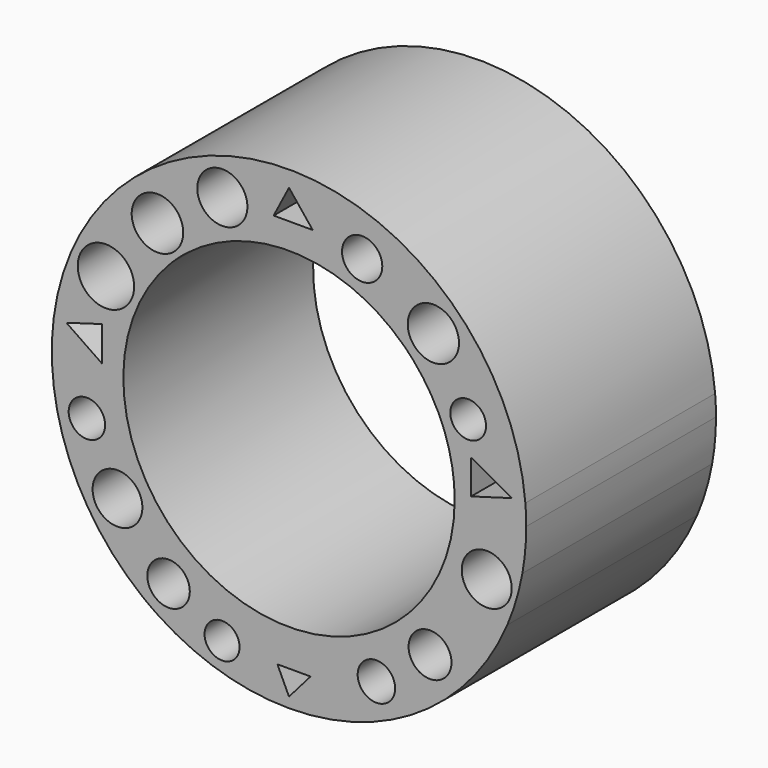
from build123d import *

# Parameters (mm, degrees)
F0_R     = 2.8256485239
F0_R_2   = 3.5765465122
F0_R_3   = 2.7439429232
F0_R_4   = 3.3466336439
F0_R_5   = 3.4276298102
F0_R_6   = 3.6294104123
F0_R_7   = 2.635041669
F0_R_8   = 2.702327646
F0_R_9   = 2.972249944
F0_R_10  = 2.6404432644
F0_R_11  = 2.6241403427
F0_R_12  = 2.7159497561
F0_R_13  = 2.2390207397
F0_R_14  = 2.2607819858
F0_R_15  = 1.9741758504
F0_R_16  = 2.1219308593
F0_R_17  = 1.8827842167
F0_R_18  = 1.845321618
F0_R_19  = 1.9213841029
F1_DEPTH = 25


with BuildPart() as f1:
    # F0 (on Front) → F1 (new body)
    with BuildSketch(Plane.XZ):
        with BuildLine():
            ThreePointArc((24.5960952758, -4.4757230907), (24.8988190673, -2.2469555075), (25, 0))
            ThreePointArc((25, 0), (24.9769503507, 1.073289886), (24.9078439057, 2.1446006555))
            ThreePointArc((24.9078439057, 2.1446006555), (0.5208838947, 24.9945730103), (-24.7968706797, 3.1804409279))
            ThreePointArc((-24.7968706797, 3.1804409279), (-23.1514874221, -9.4344385176), (-15.5110739298, -19.6062894384))
            ThreePointArc((-15.5110739298, -19.6062894384), (-13.7709472228, -14.2438804489), (-9.2095510788, -17.5570566207))
            ThreePointArc((-9.2095510788, -17.5570566207), (-10.6398306506, -20.3713740635), (-13.7563172666, -20.8749547368))
            ThreePointArc((-13.7563172666, -20.8749547368), (-7.1807427047, -23.9465432622), (0, -25))
            ThreePointArc((0, -25), (13.7903970721, -20.8524566561), (23.0050925772, -9.7859958876))
            ThreePointArc((23.0050925772, -9.7859958876), (16.860220208, -5.0514647504), (24.5960952758, -4.4757230907))
        make_face()
        with Locations((-7.0527321659, -21.0157949477)):
            Circle(F0_R, mode=Mode.SUBTRACT)
        with Locations((-18.0755164474, -11.404263787)):
            Circle(F0_R_2, mode=Mode.SUBTRACT)
        with Locations((-21.2986432016, -5.0265877508)):
            Circle(F0_R_3, mode=Mode.SUBTRACT)
        Polygon((4.266737029, -20.0934484601), (0, -25), (-2.6190390345, -20.0934484601), align=None, mode=Mode.SUBTRACT)
        with Locations((9.209163487, -19.5164699107)):
            Circle(F0_R_4, mode=Mode.SUBTRACT)
        with Locations((14.8604605347, -15.1914991438)):
            Circle(F0_R_5, mode=Mode.SUBTRACT)
        with BuildLine():
            Line((-18.9121421427, -0.7938772906), (-24.7968706797, 3.1804409279))
            Line((-24.7968706797, 3.1804409279), (-19.3468905014, 5.0684465431))
            ThreePointArc((-19.3468905014, 5.0684465431), (-21.9186154294, 11.469459375), (-15.5548330751, 8.8069401681))
            ThreePointArc((-15.5548330751, 8.8069401681), (-16.5182971087, 6.3016908172), (-18.9121421427, 5.0875890061))
            Line((-18.9121421427, 5.0875890061), (-18.9121421427, -0.7938772906))
        make_face(mode=Mode.SUBTRACT)
        with Locations((-7.0253848098, 20.105432719)):
            Circle(F0_R_6, mode=Mode.SUBTRACT)
        with BuildLine():
            Line((19.5046194307, 4.8279847044), (24.9078439057, 2.1446006555))
            Line((24.9078439057, 2.1446006555), (18.717167899, 0))
            Line((18.717167899, 0), (18.717167899, 4.7704775792))
            ThreePointArc((18.717167899, 4.7704775792), (17.4488389654, 5.1069570809), (16.4242905584, 5.9268212774))
            ThreePointArc((16.4242905584, 5.9268212774), (17.1998275024, 3.0083990244), (17.4609430101, 0))
            ThreePointArc((17.4609430101, 0), (-6.6059492578, -16.1631050607), (-12.4625227562, 12.2298837833))
            ThreePointArc((-12.4625227562, 12.2298837833), (-16.8312529103, 17.4566617233), (-10.3065616702, 15.4987508431))
            ThreePointArc((-10.3065616702, 15.4987508431), (-10.4242678564, 14.5913936768), (-10.7695943307, 13.7441030538))
            ThreePointArc((-10.7695943307, 13.7441030538), (-2.5101792072, 17.2795697617), (6.4137999623, 16.2403109836))
            ThreePointArc((6.4137999623, 16.2403109836), (5.9393579148, 21.9051948536), (10.9397131516, 19.2010402679))
            ThreePointArc((10.9397131516, 19.2010402679), (9.558784183, 16.551960716), (6.5962795119, 16.1670537638))
            ThreePointArc((6.5962795119, 16.1670537638), (9.4231129686, 14.6999820674), (11.9364463054, 12.7438526513))
            ThreePointArc((11.9364463054, 12.7438526513), (14.1879258767, 18.3986934482), (19.0337079573, 14.7156538442))
            ThreePointArc((19.0337079573, 14.7156538442), (17.0365778867, 11.3571292026), (13.1320353046, 11.5080050208))
            ThreePointArc((13.1320353046, 11.5080050208), (14.5572332623, 9.6421725015), (15.7192265164, 7.6020029287))
            ThreePointArc((15.7192265164, 7.6020029287), (18.7083751896, 11.1226574982), (22.0615752041, 7.9468004405))
            ThreePointArc((22.0615752041, 7.9468004405), (21.3406257649, 5.9303038237), (19.5046194307, 4.8279847044))
        make_face(mode=Mode.SUBTRACT)
        Polygon((3.975788597, 19.6694843471), (-2.6190390345, 19.6694843471), (0, 24.2276750505), align=None, mode=Mode.SUBTRACT)
        with BuildLine():
            ThreePointArc((23.0050925772, -9.7859958876), (23.9482362722, -7.1750943862), (24.5960952758, -4.4757230907))
            ThreePointArc((24.5960952758, -4.4757230907), (16.860220208, -5.0514647504), (23.0050925772, -9.7859958876))
        make_face()
        with Locations((20.8382867277, -6.2433271669)):
            Circle(F0_R_7, mode=Mode.SUBTRACT)
        with BuildLine():
            ThreePointArc((11.9364463054, 12.7438526513), (12.5494630323, 12.1406551883), (13.1320353046, 11.5080050208))
            ThreePointArc((13.1320353046, 11.5080050208), (17.0365778867, 11.3571292026), (19.0337079573, 14.7156538442))
            ThreePointArc((19.0337079573, 14.7156538442), (14.1879258767, 18.3986934482), (11.9364463054, 12.7438526513))
        make_face()
        with Locations((15.2111686766, 14.7156538442)):
            Circle(F0_R_8, mode=Mode.SUBTRACT)
        with BuildLine():
            ThreePointArc((-15.5548330751, 8.8069401681), (-21.9186154294, 11.469459375), (-19.3468905014, 5.0684465431))
            Line((-19.3468905014, 5.0684465431), (-18.9121421427, 5.2190539427))
            Line((-18.9121421427, 5.2190539427), (-18.9121421427, 5.0875890061))
            ThreePointArc((-18.9121421427, 5.0875890061), (-16.5182971087, 6.3016908172), (-15.5548330751, 8.8069401681))
        make_face()
        with Locations((-19.2937050015, 8.8069401681)):
            Circle(F0_R_9, mode=Mode.SUBTRACT)
        with Locations((-7.0253848098, 20.105432719)):
            Circle(F0_R_6)
        with Locations((-7.0253848098, 20.105432719)):
            Circle(F0_R_10, mode=Mode.SUBTRACT)
        with Locations((-18.0755164474, -11.404263787)):
            Circle(F0_R_2)
        with Locations((-18.0755164474, -11.404263787)):
            Circle(F0_R_11, mode=Mode.SUBTRACT)
        with BuildLine():
            ThreePointArc((-10.3065616702, 15.4987508431), (-16.8312529103, 17.4566617233), (-12.4625227562, 12.2298837833))
            ThreePointArc((-12.4625227562, 12.2298837833), (-11.6407057812, 13.0145495395), (-10.7695943307, 13.7441030538))
            ThreePointArc((-10.7695943307, 13.7441030538), (-10.4242678564, 14.5913936768), (-10.3065616702, 15.4987508431))
        make_face()
        with Locations((-13.8626694679, 15.4987508431)):
            Circle(F0_R_12, mode=Mode.SUBTRACT)
        with BuildLine():
            ThreePointArc((-9.2095510788, -17.5570566207), (-13.7709472228, -14.2438804489), (-15.5110739298, -19.6062894384))
            ThreePointArc((-15.5110739298, -19.6062894384), (-14.6474374814, -20.2596291977), (-13.7563172666, -20.8749547368))
            ThreePointArc((-13.7563172666, -20.8749547368), (-10.6398306506, -20.3713740635), (-9.2095510788, -17.5570566207))
        make_face()
        with Locations((-12.6935141161, -17.5570566207)):
            Circle(F0_R_13, mode=Mode.SUBTRACT)
        with Locations((14.8604605347, -15.1914991438)):
            Circle(F0_R_5)
        with Locations((14.8604605347, -15.1914991438)):
            Circle(F0_R_14, mode=Mode.SUBTRACT)
        with Locations((9.209163487, -19.5164699107)):
            Circle(F0_R_4)
        with Locations((9.209163487, -19.5164699107)):
            Circle(F0_R_15, mode=Mode.SUBTRACT)
        with BuildLine():
            ThreePointArc((6.4137999623, 16.2403109836), (6.5051428606, 16.2039392484), (6.5962795119, 16.1670537638))
            ThreePointArc((6.5962795119, 16.1670537638), (9.558784183, 16.551960716), (10.9397131516, 19.2010402679))
            ThreePointArc((10.9397131516, 19.2010402679), (5.9393579148, 21.9051948536), (6.4137999623, 16.2403109836))
        make_face()
        with Locations((7.7083422802, 19.2010402679)):
            Circle(F0_R_16, mode=Mode.SUBTRACT)
        with BuildLine():
            Line((18.717167899, 5.2190539427), (19.5046194307, 4.8279847044))
            ThreePointArc((19.5046194307, 4.8279847044), (21.3406257649, 5.9303038237), (22.0615752041, 7.9468004405))
            ThreePointArc((22.0615752041, 7.9468004405), (18.7083751896, 11.1226574982), (15.7192265164, 7.6020029287))
            ThreePointArc((15.7192265164, 7.6020029287), (16.0935695505, 6.7735920991), (16.4242905584, 5.9268212774))
            ThreePointArc((16.4242905584, 5.9268212774), (17.4488389654, 5.1069570809), (18.717167899, 4.7704775792))
            Line((18.717167899, 4.7704775792), (18.717167899, 5.2190539427))
        make_face()
        with Locations((18.8810285181, 7.9468004405)):
            Circle(F0_R_17, mode=Mode.SUBTRACT)
        with Locations((-7.0527321659, -21.0157949477)):
            Circle(F0_R)
        with Locations((-7.0527321659, -21.0157949477)):
            Circle(F0_R_18, mode=Mode.SUBTRACT)
        with Locations((-21.2986432016, -5.0265877508)):
            Circle(F0_R_3)
        with Locations((-21.2986432016, -5.0265877508)):
            Circle(F0_R_19, mode=Mode.SUBTRACT)
        with BuildLine():
            Line((-19.3468905014, 5.0684465431), (-24.7968706797, 3.1804409279))
            Line((-24.7968706797, 3.1804409279), (-18.9121421427, -0.7938772906))
            Line((-18.9121421427, -0.7938772906), (-18.9121421427, 5.0875890061))
            ThreePointArc((-18.9121421427, 5.0875890061), (-19.1292375855, 5.0716873319), (-19.3468905014, 5.0684465431))
        make_face()
        Polygon((-19.7024215013, 4.2425552383), (-19.7024215013, 0.5726945819), (-23.453835398, 3.1415971462), align=None, mode=Mode.SUBTRACT)
        Polygon((-2.6190390345, -20.0934484601), (0, -25), (4.266737029, -20.0934484601), align=None)
        Polygon((0, -23.921410939), (-1.2212268775, -21.310839802), (2.2701525595, -21.310839802), align=None, mode=Mode.SUBTRACT)
        with BuildLine():
            Line((18.717167899, 0), (24.9078439057, 2.1446006555))
            Line((24.9078439057, 2.1446006555), (19.5046194307, 4.8279847044))
            ThreePointArc((19.5046194307, 4.8279847044), (19.1126850593, 4.774701377), (18.717167899, 4.7704775792))
            Line((18.717167899, 4.7704775792), (18.717167899, 0))
        make_face()
        Polygon((23.5085282475, 2.1446006555), (19.1881656647, 0.9002434672), (19.1881656647, 4.50054463), align=None, mode=Mode.SUBTRACT)
        Polygon((0, 24.2276750505), (-2.6190390345, 19.6694843471), (3.975788597, 19.6694843471), align=None)
        Polygon((2.4991026148, 20.1859623194), (-1.6240375116, 20.1859623194), (0, 23.2999436557), align=None, mode=Mode.SUBTRACT)
        with BuildLine():
            ThreePointArc((18.717167899, 4.7704775792), (19.1126850593, 4.774701377), (19.5046194307, 4.8279847044))
            Line((19.5046194307, 4.8279847044), (18.717167899, 5.2190539427))
            Line((18.717167899, 5.2190539427), (18.717167899, 4.7704775792))
        make_face()
        with BuildLine():
            Line((-18.9121421427, 5.2190539427), (-19.3468905014, 5.0684465431))
            ThreePointArc((-19.3468905014, 5.0684465431), (-19.1292375855, 5.0716873319), (-18.9121421427, 5.0875890061))
            Line((-18.9121421427, 5.0875890061), (-18.9121421427, 5.2190539427))
        make_face()
    extrude(amount=F1_DEPTH)


solid = f1.part
